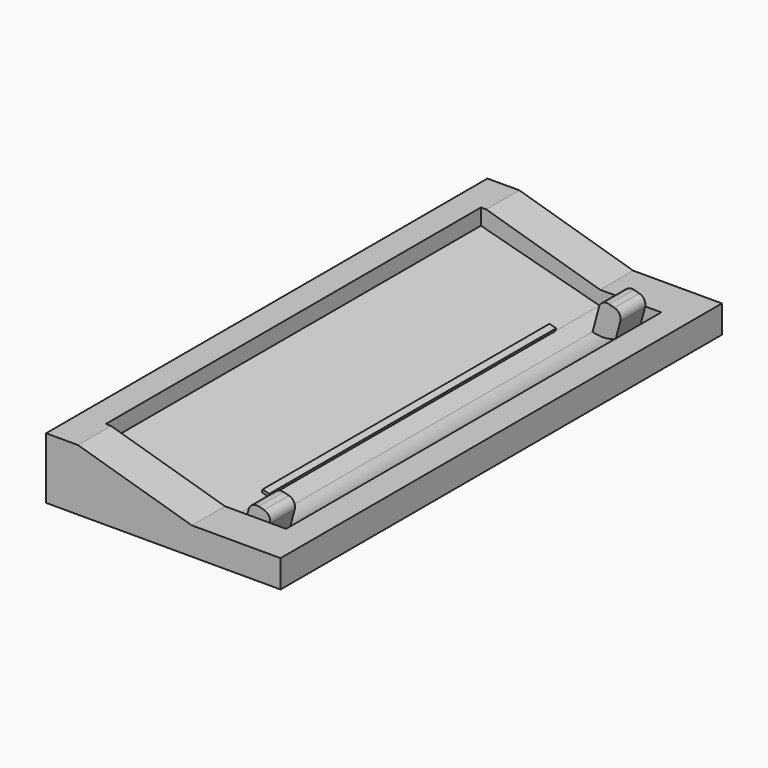
from build123d import *

# Parameters (mm, degrees)
F0_W        = 21.59
F0_H        = 50.8
F1_DEPTH    = 2.54
F3_DEPTH    = 21.59
F5_DEPTH    = 21.59
F6_T1_DEPTH = 46.99
F6_T3_DEPTH = 43.18
F7_W        = 5.334
F7_H        = 5.212301854
F8_DEPTH    = 18.7325
F10_DEPTH   = 50.8
F12_DEPTH   = 21.59
F14_DEPTH   = 16.51


# Not quite as in the source:
# - a fillet or chamfer that OpenCascade refuses, or shapes differently, is made with other operations: its cross-section is extruded or revolved along the edge and cut away or added


with BuildPart() as f1:
    # F0 (on Top) → F1 (new body)
    with BuildSketch(Plane.XY):
        with Locations((10.795, 0)):
            Rectangle(F0_W, F0_H)
    extrude(amount=F1_DEPTH)

    # F2 (on Front) → F3 (cut, symmetric)
    with BuildSketch(Plane.XZ):
        with BuildLine():
            Line((19.05, 2.54), (13.716, 2.54))
            Line((13.716, 2.54), (13.3675778015, 1.2396706526))
            Line((13.3675778015, 1.2396706526), (15.0113903727, 0.7992124017))
            ThreePointArc((15.0113903727, 0.7992124017), (17.3330984682, 0.9680336444), (19.05, 2.54))
        make_face()
    extrude(amount=F3_DEPTH, both=True, mode=Mode.SUBTRACT)

    # F4 (on Front) → F5 (join, symmetric)
    with BuildSketch(Plane.XZ):
        Polygon((15.8002708221, 3.7433543202), (15.0113903727, 0.7992124017), (16.9741516517, 0.273292102), (17.7630321012, 3.2174340206), align=None)
    extrude(amount=F5_DEPTH, both=True)

    # F6: fillet of radius 0.762 on 2 edges, made by hand

    # F6_s2 → F6_t1 (cut)
    with BuildSketch(Plane.XZ.offset(-23.495)):
        with BuildLine():
            ThreePointArc((16.5363063018, 3.5461342079), (15.9580861894, 3.4700100859), (15.6030507098, 3.0073188406))
            Line((15.6030507098, 3.0073188406), (15.8002708221, 3.7433543202))
            Line((15.8002708221, 3.7433543202), (16.5363063018, 3.5461342079))
        make_face()
    extrude(amount=F6_T1_DEPTH, mode=Mode.SUBTRACT)

    # F6_s4 → F6_t3 (cut)
    with BuildSketch(Plane.XZ.offset(-21.59)):
        with BuildLine():
            ThreePointArc((17.5658119888, 2.4813985409), (17.4896878668, 3.0596186533), (17.0269966215, 3.4146541329))
            Line((17.0269966215, 3.4146541329), (17.7630321012, 3.2174340206))
            Line((17.7630321012, 3.2174340206), (17.5658119888, 2.4813985409))
        make_face()
    extrude(amount=F6_T3_DEPTH, mode=Mode.SUBTRACT)

    # F7 (on Front) → F8 (cut, symmetric)
    with BuildSketch(Plane.XZ):
        with BuildLine():
            Line((19.05, 2.54), (13.716, 2.54))
            Line((13.716, 2.54), (13.3675778015, 1.2396706526))
            Line((13.3675778015, 1.2396706526), (15.0113903727, 0.7992124017))
            ThreePointArc((15.0113903727, 0.7992124017), (17.3330984682, 0.9680336444), (19.05, 2.54))
        make_face()
        with Locations((16.383, 5.146150927)):
            Rectangle(F7_W, F7_H)
    extrude(amount=F8_DEPTH, both=True, mode=Mode.SUBTRACT)

    # F9 (on face) → F10 (join)
    with BuildSketch(Plane.XZ.offset(25.4)):
        Polygon((0, 2.54), (13.4194806689, 2.54), (2.9378255369, 5.6436832687), (0, 5.6436832687), align=None)
    extrude(amount=-F10_DEPTH)

    # F11 (on Front) → F12 (cut, symmetric)
    with BuildSketch(Plane.XZ):
        Polygon((2.4497181869, 4.1651023194), (15.0113903727, 0.7992124017), (15.0113903727, 10.927637258), (2.4497181869, 10.927637258), align=None)
    extrude(amount=F12_DEPTH, both=True, mode=Mode.SUBTRACT)

    # F13 (on Front) → F14 (join, symmetric)
    with BuildSketch(Plane.XZ):
        Polygon((12.7542149018, 1.4040207463), (13.3675778015, 1.2396706526), (13.4333178389, 1.4850158125), (12.8199549392, 1.6493659062), align=None)
    extrude(amount=F14_DEPTH, both=True)


solid = f1.part
